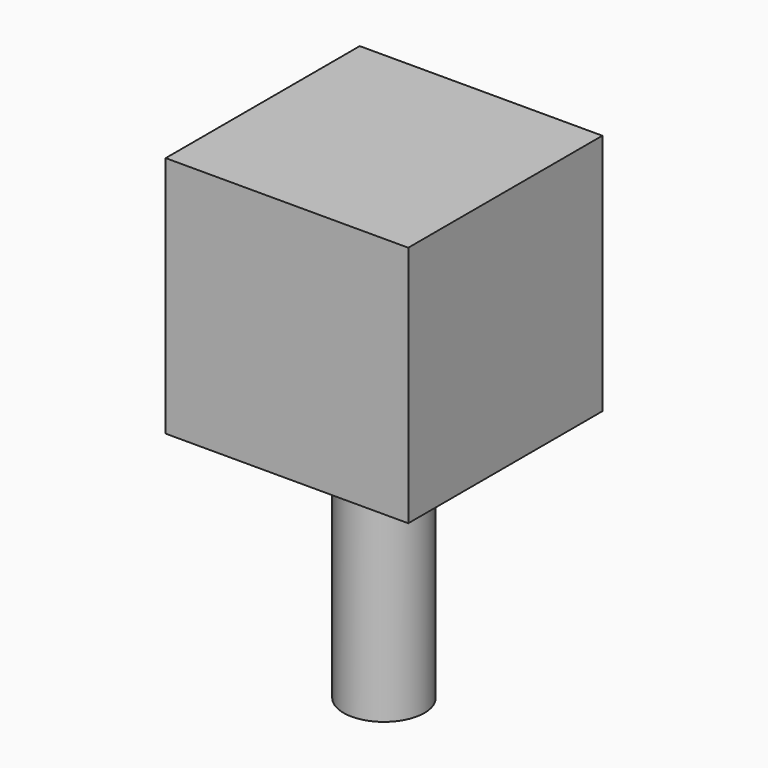
from build123d import *

# Parameters (mm, degrees)
F0_W     = 30
F0_H     = 30
F1_DEPTH = 30
F2_R     = 5
F3_DEPTH = 30
F4_R     = 2.5
F5_DEPTH = 70


with BuildPart() as f1:
    # F0 (on Top) → F1 (new body)
    with BuildSketch(Plane.XY):
        Rectangle(F0_W, F0_H)
    extrude(amount=F1_DEPTH)


with BuildPart() as f3:
    # F2 (on Top) → F3 (new body)
    with BuildSketch(Plane.XY):
        Circle(F2_R)
    extrude(amount=-F3_DEPTH)

    # F4 (on face) → F5 (cut)
    with BuildSketch(Plane(origin=(0, 0, -30), x_dir=(1, 0, 0), z_dir=(0, 0, -1))):
        Circle(F4_R)
    extrude(amount=-F5_DEPTH, mode=Mode.SUBTRACT)


solid = Compound([f1.part, f3.part])
